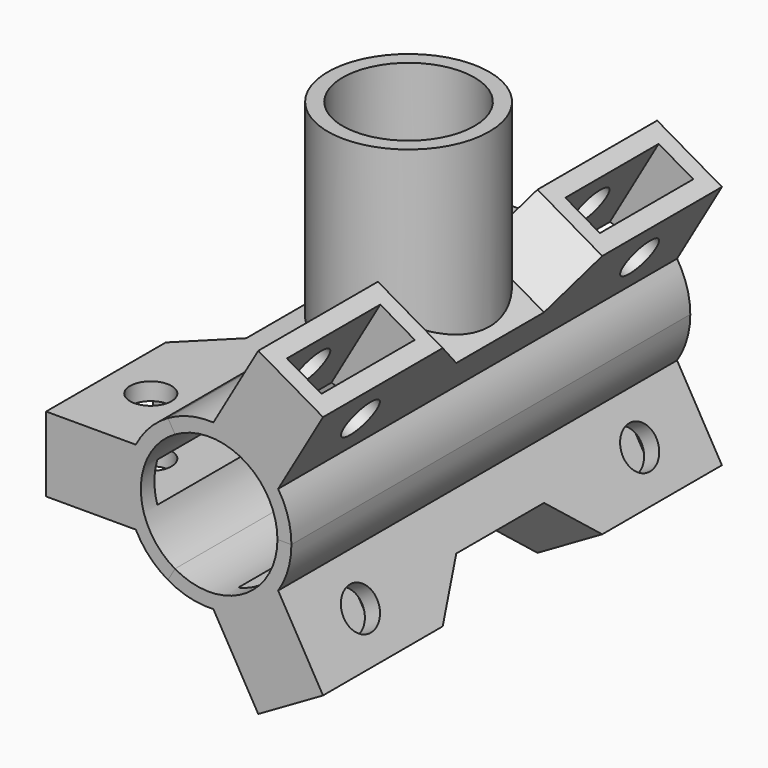
from build123d import *
from build123d import SkipClean  # not in build123d's __all__

# Parameters (mm, degrees)
F0_R      = 4.16
F1_DEPTH  = 15
F3_DEPTH  = 100
F4_W      = 23.4
F4_H      = 8
F5_DEPTH  = 25
F7_COUNT  = 3
F9_START  = 22
F8_R      = 16.208
F8_R_2    = 13.208
F9_DEPTH  = 38
F10_R     = 12.7
F11_DEPTH = 40
F12_R     = 13.208
F13_DEPTH = 40


# Not quite as in the source:
# - a feature names something its author has since deleted; it is built from what else it names


with BuildPart() as f1:
    # F0 (on Top) → F1 (new body)
    with BuildSketch(Plane.XY):
        Polygon((-32.7, 0), (-14.7, 0), (-14.7, 50), (-14.7, 100), (-32.7, 100), (-32.7, 70), (-23.7483102828, 61), (-23.7483102828, 50), (-23.7483102828, 39), (-32.7, 30), align=None)
        with Locations((-23.7, 15)):
            Circle(F0_R, mode=Mode.SUBTRACT)
        with Locations((-23.7, 85)):
            Circle(F0_R, mode=Mode.SUBTRACT)
    extrude(amount=F1_DEPTH)

    # F2 (on face) → F3 (join)
    with BuildSketch(Plane.XZ):
        with BuildLine():
            Line((-14.7, 0), (-14.7, 15))
            ThreePointArc((-14.7, 15), (-16.5027270474, 7.5), (-14.7, 0))
        make_face()
        with BuildLine():
            ThreePointArc((-6.85, -4.3645480318), (-13.7, 7.5), (-6.85, 19.3645480318))
            Line((-6.85, 19.3645480318), (-8.2513635237, 21.7917808547))
            ThreePointArc((-8.2513635237, 21.7917808547), (-11.9675955686, 18.8629510386), (-14.7, 15))
            Line((-14.7, 15), (-14.7, 0))
            ThreePointArc((-14.7, 0), (-11.9675955686, -3.8629510386), (-8.2513635237, -6.7917808547))
            Line((-8.2513635237, -6.7917808547), (-6.85, -4.3645480318))
        make_face()
    extrude(amount=-F3_DEPTH)

    # F4 (on face) → F5 (cut)
    with BuildSketch(Plane(origin=(-32.7, 0, 0), x_dir=(0, -1, 0), z_dir=(-1, 0, 0))):
        with Locations((-84.9, 7.5)):
            Rectangle(F4_W, F4_H)
        with Locations((-15.1, 7.5)):
            Rectangle(F4_W, F4_H)
    extrude(amount=-F5_DEPTH, mode=Mode.SUBTRACT)

    # F7: F1 ×3 about axis
    f7_axis = Axis((0, 0, 7.5), (0, -1, 0))


with BuildPart() as f1_1:
    add(f1.part, clean=False)
    with SkipClean():  # cleaning this boolean's faces spoils the solid; the shape is the same uncleaned
        for i in range(1, F7_COUNT):
            add(f1.part.rotate(f7_axis, i * 360 / F7_COUNT), clean=False)

    # F8 (on Top) → F9 (join)
    with BuildSketch(Plane.XY.offset(F9_START)):
        with Locations((0, 50)):
            Circle(F8_R)
        with Locations((0, 50)):
            Circle(F8_R_2, mode=Mode.SUBTRACT)
    with SkipClean():  # cleaning this boolean's faces spoils the solid; the shape is the same uncleaned
        extrude(amount=F9_DEPTH)

    # F10 (on face) → F11 (cut)
    with BuildSketch(Plane.XY.offset(60)):
        with Locations((0, 50)):
            Circle(F10_R)
    with SkipClean():  # cleaning this boolean's faces spoils the solid; the shape is the same uncleaned
        extrude(amount=-F11_DEPTH, mode=Mode.SUBTRACT)

    # F12 (on face) → F13 (cut)
    with BuildSketch(Plane.XY.offset(60)):
        with Locations((0, 50)):
            Circle(F12_R)
    with SkipClean():  # cleaning this boolean's faces spoils the solid; the shape is the same uncleaned
        extrude(amount=-F13_DEPTH, mode=Mode.SUBTRACT)


solid = f1_1.part
